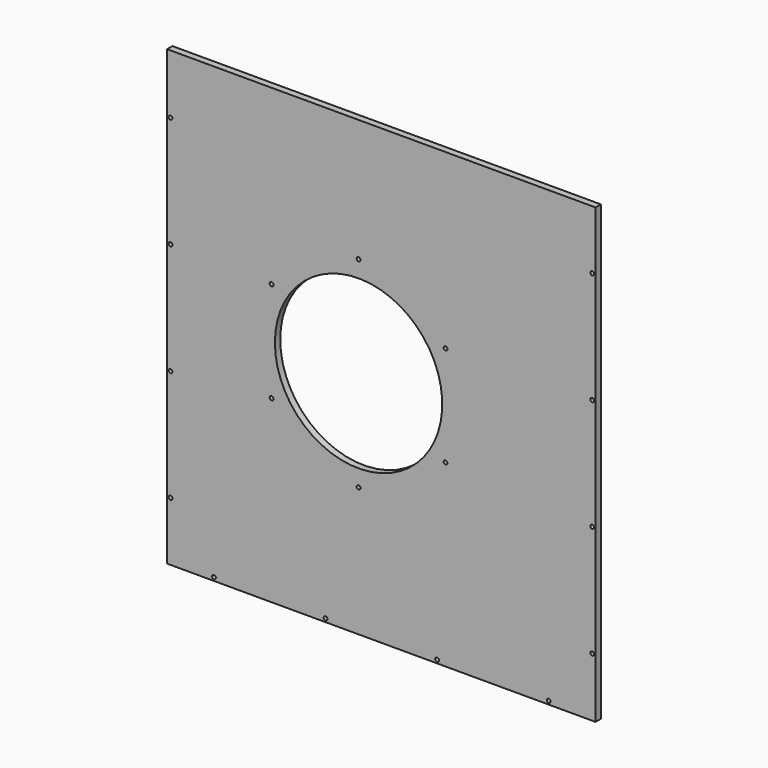
from build123d import *

# Parameters (mm, degrees)
F0_W     = 384
F0_H     = 406
F2_DEPTH = 6
F3_D     = 3.4
F5_D     = 3.4
F4_R     = 75
F6_DEPTH = 6
F8_D     = 3.4
F9_D     = 3.4
F10_D    = 3.4


# Not quite as in the source:
# - a feature names something its author has since deleted; it is built from what else it names


with BuildPart() as f2:
    # F0 (on Front) → F2 (new body)
    with BuildSketch(Plane.XZ):
        Rectangle(F0_W, F0_H)
    extrude(amount=F2_DEPTH)

    # F3 (through all)
    with Locations(Plane(origin=(0, 0, 0), x_dir=(1, 0, 0), z_dir=(0, 1, 0))):
        with Locations((189, -150), (189, -50), (189, 150), (150, 200), (-50, 200), (-150, 200), (-189, -50), (-189, -150), (-189, 50)):
            Hole(F3_D / 2)

    # F5 (through all)
    with Locations(Plane(origin=(0, 0, 0), x_dir=(-1, 0, 0), z_dir=(0, 1, 0))):
        with Locations((98.3422863406, 48), (20.4, -87), (-57.5422863406, 48), (98.3422863406, -42), (20.4, 93), (-57.5422863406, -42)):
            Hole(F5_D / 2)


with BuildPart() as f6:
    # F4 (on face) → F6 (new body)
    with BuildSketch(Plane(origin=(0, 0, 0), x_dir=(-1, 0, 0), z_dir=(0, 1, 0))):
        with Locations((20.4, 3)):
            Circle(F4_R)
    extrude(amount=-F6_DEPTH)


with BuildPart() as f2_1:
    add(f2.part)

    # F7: cut F6
    add(f6.part, mode=Mode.SUBTRACT)

    # F8 (through all)
    with Locations(Plane(origin=(0, 0, 0), x_dir=(1, 0, 0), z_dir=(0, 1, 0))):
        with Locations((-189, 150)):
            Hole(F8_D / 2)

    # F9 (through all)
    with Locations(Plane(origin=(0, 0, 0), x_dir=(1, 0, 0), z_dir=(0, 1, 0))):
        with Locations((189, 50)):
            Hole(F9_D / 2)

    # F10 (through all)
    with Locations(Plane(origin=(0, 0, 0), x_dir=(1, 0, 0), z_dir=(0, 1, 0))):
        with Locations((50, 200)):
            Hole(F10_D / 2)


solid = f2_1.part
